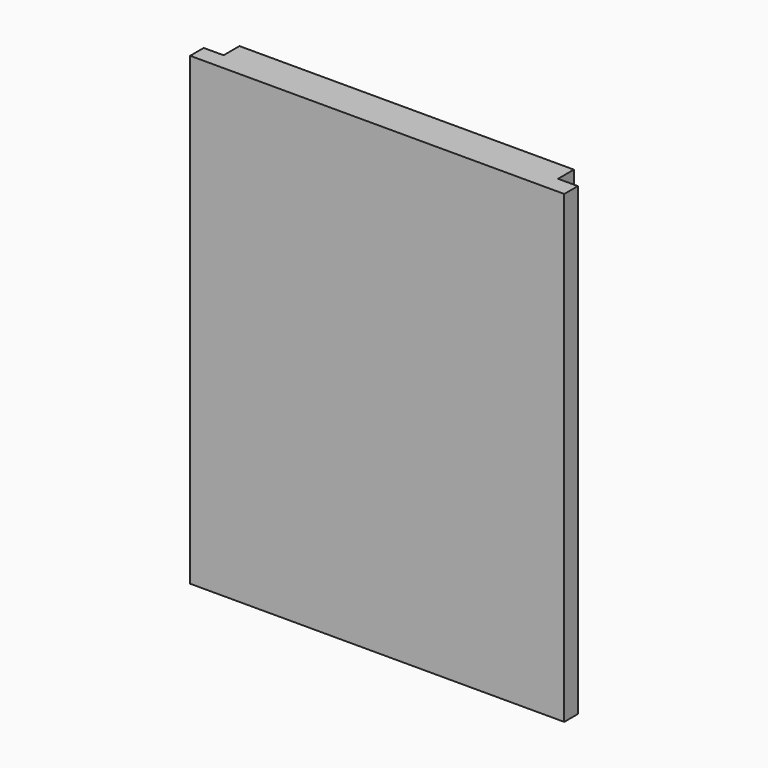
from build123d import *

# Parameters (mm, degrees)
F0_W     = 209.55
F0_H     = 20.6375
F1_DEPTH = 260.35
F2_W     = 209.55
F2_H     = 22.225
F3_DEPTH = 11.1125
F4_W     = 11.1125
F4_H     = 11.1125
F5_DEPTH = 260.351


# Not quite as in the source:
# - a length typed as a fraction of an inch, garbled in the dataset ("3 / 203.2 mm" for 3/8 in), is restored


with BuildPart() as f1:
    # F0 (on Top) → F1 (new body)
    with BuildSketch(Plane.XY):
        with Locations((0, 10.31875)):
            Rectangle(F0_W, F0_H)
    extrude(amount=-F1_DEPTH)

    # F2 (on face) → F3 (cut)
    with BuildSketch(Plane(origin=(0, 20.6375, 0), x_dir=(-1, 0, 0), z_dir=(0, 1, 0))):
        with Locations((0, -239.7125)):
            Rectangle(F2_W, F2_H)
    extrude(amount=-F3_DEPTH, mode=Mode.SUBTRACT)

    # F4 (on face) → F5 (cut, through all)
    with BuildSketch(Plane(origin=(0, 0, -260.35), x_dir=(1, 0, 0), z_dir=(0, 0, -1))):
        with Locations((-99.21875, -15.08125)):
            Rectangle(F4_W, F4_H)
        with Locations((99.21875, -15.08125)):
            Rectangle(F4_W, F4_H)
    extrude(amount=-F5_DEPTH, mode=Mode.SUBTRACT)


solid = f1.part
